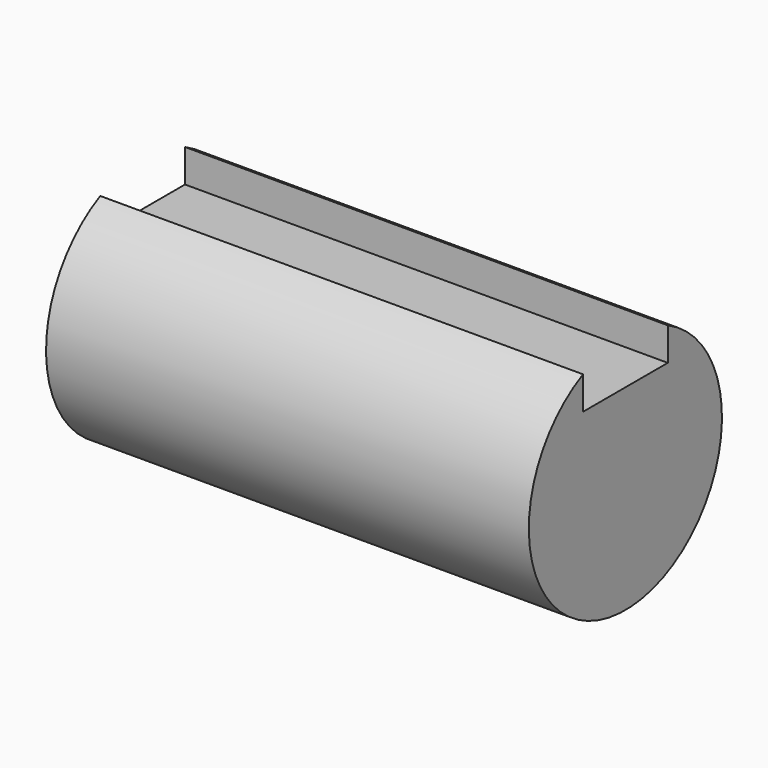
from build123d import *

# Parameters (mm, degrees)
F3_D         = 6.7564
F3_DEPTH     = 5.08
F3_TIP       = 2.0298273432
F6_TEXT_SIZE = 30.7580883726
F7_DEPTH     = 1.27
F9_DEPTH     = 12.7


# Not quite as in the source:
# - Text() gives the source's letters only with a copy of the font that has no kerning and outlines rounded to 1/6400 em; it was checked with that copy


with BuildPart() as f1:
    # F0 (on Front) → F1 (revolve)
    with BuildSketch(Plane.XZ):
        with BuildLine():
            Line((-11.938, 0), (0, 0))
            Line((0, 0), (0, 26.4740031074))
            ThreePointArc((0, 26.4740031074), (-2.1693802982, 29.9126753794), (-6.2070692882, 29.4354485024))
            add(Edge.make_bspline(
                [(-6.2070692882, 29.4354485024), (-11.938, 24.7966872998), (-11.938, 15.875)],
                knots=[3.6883758692, 3.6883758692, 3.6883758692, 4.7123889804, 4.7123889804, 4.7123889804], degree=2, weights=[1, 0.8717631966, 1]))
            Line((-11.938, 15.875), (-11.938, 0))
        make_face()
    revolve(axis=Axis((-5.969, 0, 0), (-1, 0, 0)))

    # F3
    with Locations(Plane.YZ):
        with Locations((0, 0)):
            Hole(F3_D / 2, depth=F3_DEPTH)
            with Locations((0, 0, -(F3_DEPTH + F3_TIP / 2))):  # 118° drill point
                Cone(0, F3_D / 2, F3_TIP, mode=Mode.SUBTRACT)

    # F4 (on face) → F5 (join, up to the next surface of F1)
    with BuildSketch(Plane.YZ):
        with BuildLine():
            Line((-1.190625, 2.187575), (1.190625, 2.187575))
            Line((1.190625, 2.187575), (1.190625, 3.1614312185))
            ThreePointArc((1.190625, 3.1614312185), (0, 3.3782), (-1.190625, 3.1614312185))
            Line((-1.190625, 3.1614312185), (-1.190625, 2.187575))
        make_face()
    extrude(until=Until.NEXT, dir=(-1, 0, 0))

    # F6 (on face) → F7 (cut)
    with BuildSketch(Plane(origin=(-11.938, 0, 0), x_dir=(0, -1, 0), z_dir=(-1, 0, 0))):
        with Locations((-11.3756867466, -11.0729118142)):
            Text('H', F6_TEXT_SIZE, font='Open Sans', font_style=FontStyle.BOLD, text_align=(TextAlign.LEFT, TextAlign.BOTTOM))
    extrude(amount=-F7_DEPTH, mode=Mode.SUBTRACT)


with BuildPart() as f9:
    # F8 (on face) → F9 (new body)
    with BuildSketch(Plane.YZ):
        with BuildLine():
            Line((-1.393825, 1.984375), (-1.393825, 2.8526964208))
            ThreePointArc((-1.393825, 2.8526964208), (0, -3.175), (1.393825, 2.8526964208))
            Line((1.393825, 2.8526964208), (1.393825, 1.984375))
            Line((1.393825, 1.984375), (-1.393825, 1.984375))
        make_face()
    extrude(amount=F9_DEPTH)


solid = f9.part
